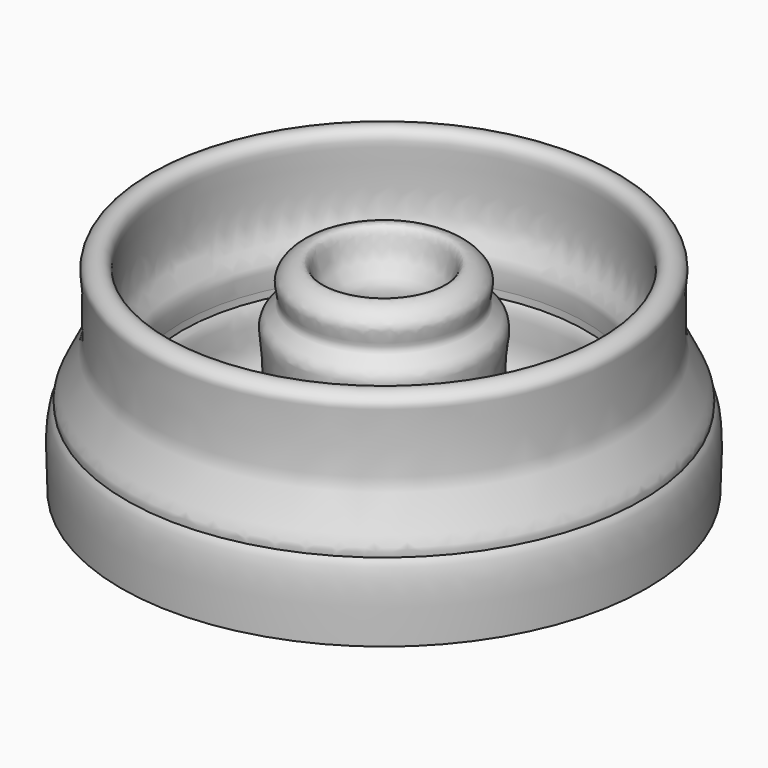
from build123d import *


with BuildPart() as f1:
    # F0 (on Front) → F1 (revolve)
    with BuildSketch(Plane.XZ):
        with BuildLine():
            add(Edge.make_bspline(
                [(-5.5100140162, 0), (-7.4768554599, 1.6512499989), (-8.4868156211, 11.2822794795), (-11.6145699642, 16.211100514), (-14.0046197921, 17.3335876316)],
                knots=[0.0567445852, 0.0567445852, 0.0567445852, 0.0567445852, 0.1379704075, 0.2072796019, 0.2072796019, 0.2072796019, 0.2072796019], degree=3))
            add(Edge.make_bspline(
                [(-14.0046197921, 17.3335876316), (-16.264658586, 18.3950150553), (-19.3741295412, 18.430981238), (-21.3513057679, 17.5631716847)],
                knots=[0.2072796019, 0.2072796019, 0.2072796019, 0.2072796019, 0.2728185988, 0.2728185988, 0.2728185988, 0.2728185988], degree=3))
            add(Edge.make_bspline(
                [(-21.3513057679, 17.5631716847), (-22.9378846487, 16.8668006222), (-24.856551537, 14.0064203945), (-25.3428790843, 6.7308083338), (-27.5189999089, 1.7281130761), (-30.8207862539, 0.4264153255), (-32.6009168711, 1.22e-08)],
                knots=[0.2728185988, 0.2728185988, 0.2728185988, 0.2728185988, 0.3254101619, 0.390496916, 0.4452692569, 0.4997726035, 0.4997726035, 0.4997726035, 0.4997726035], degree=3))
            add(Edge.make_bspline(
                [(-32.6009168435, 0), (-23.5706158992, 0), (-14.5403149549, 0), (-5.5100140107, 0)],
                knots=[25.9429850471, 25.9429850471, 25.9429850471, 25.9429850471, 53.0338878798, 53.0338878798, 53.0338878798, 53.0338878798], degree=3))
        make_face()
        with BuildLine():
            add(Edge.make_bspline(
                [(-14.0046197921, 17.3335876316), (-16.264658586, 18.3950150553), (-19.3741295412, 18.430981238), (-21.3513057679, 17.5631716847)],
                knots=[0.2072796019, 0.2072796019, 0.2072796019, 0.2072796019, 0.2728185988, 0.2728185988, 0.2728185988, 0.2728185988], degree=3))
            add(Edge.make_bspline(
                [(-21.3513057679, 17.5631716847), (-21.1820220673, 21.0577877247), (-20.8801300759, 27.2899092584), (-22.6799382537, 34.1653744535), (-17.1221063441, 36.9227227126), (-20.7290149123, 42.3952693374), (-12.6347622732, 47.302902282), (-12.7254316197, 39.345986815), (-7.9522904735, 35.8953625402), (-10.1102283491, 28.7576830255), (-7.0596366051, 15.4205940348), (-12.0270388133, 16.7888635267), (-14.0046197921, 17.3335876316)],
                knots=[0, 0, 0, 0, 0.1262257386, 0.2251045993, 0.3085069257, 0.3957592528, 0.4903294159, 0.583105022, 0.673312871, 0.780958545, 0.9127970322, 1, 1, 1, 1], degree=3))
        make_face()
    revolve(axis=Axis((0, 0, 38.2831208408), (0, 0, 1)))


with BuildPart() as f1b:
    # F0 (on Front) → F1, piece 2 (revolve)
    with BuildSketch(Plane.XZ):
        with BuildLine():
            add(Edge.make_bspline(
                [(-58.5439018905, 0), (-51.7329126534, 0), (-44.9219234162, 0), (-38.1109341791, 0)],
                knots=[0, 0, 0, 0, 20.4329677115, 20.4329677115, 20.4329677115, 20.4329677115], degree=3))
            add(Edge.make_bspline(
                [(-38.1109341979, 0), (-39.7350614236, 0.6328310893), (-42.3709629032, 3.5674251118), (-44.497911567, 8.512945314), (-43.4937968549, 15.0815158027), (-44.9984520674, 16.8744195253)],
                knots=[0.5565172055, 0.5565172055, 0.5565172055, 0.5565172055, 0.6120735986, 0.6692323198, 0.7381048965, 0.7381048965, 0.7381048965, 0.7381048965], degree=3))
            add(Edge.make_bspline(
                [(-44.9984520674, 16.8744195253), (-46.4682072785, 18.6257374135), (-52.6748450805, 18.6928178626), (-56.4195166036, 18.0445218661), (-57.3959834874, 16.8744195253)],
                knots=[0.7381048965, 0.7381048965, 0.7381048965, 0.7381048965, 0.8053799955, 0.8598764036, 0.8598764036, 0.8598764036, 0.8598764036], degree=3))
            add(Edge.make_bspline(
                [(-57.3959834874, 16.8744195253), (-58.5065944281, 15.5435720761), (-58.971992813, 9.9615017872), (-58.697162445, 3.5663108174), (-58.5439018905, 0)],
                knots=[0.8598764036, 0.8598764036, 0.8598764036, 0.8598764036, 0.9218593627, 1, 1, 1, 1], degree=3))
        make_face()
        with BuildLine():
            add(Edge.make_bspline(
                [(-44.9984520674, 16.8744195253), (-46.4682072785, 18.6257374135), (-52.6748450805, 18.6928178626), (-56.4195166036, 18.0445218661), (-57.3959834874, 16.8744195253)],
                knots=[0.7381048965, 0.7381048965, 0.7381048965, 0.7381048965, 0.8053799955, 0.8598764036, 0.8598764036, 0.8598764036, 0.8598764036], degree=3))
            add(Edge.make_bspline(
                [(-44.9984520674, 18.4815078974), (-44.9984520674, 17.9458117733), (-44.9984520674, 17.4101156493), (-44.9984520674, 16.8744195253)],
                knots=[0, 0, 0, 0, 1.6070883721, 1.6070883721, 1.6070883721, 1.6070883721], degree=3))
            add(Edge.make_bspline(
                [(-57.3959834874, 16.8744195253), (-57.4715446562, 17.3499237875), (-57.6848422564, 18.6921994511), (-54.9401189391, 23.4840896745), (-51.9408575122, 29.3763854334), (-52.8208897576, 35.1752529667), (-52.2423948178, 40.8160501854), (-53.4284694884, 44.8525009993), (-49.8042473471, 46.8159805052), (-47.0898142548, 45.1735042208), (-47.5753866113, 40.3334642214), (-48.4768776708, 28.2128829532), (-44.2823912341, 24.1291973687), (-44.7602116927, 20.3605488851), (-44.9984520674, 18.4815078974)],
                knots=[0, 0, 0, 0, 0.0480091479, 0.1355224673, 0.2335006939, 0.3242294406, 0.4149581578, 0.487541167, 0.5551750374, 0.6133988864, 0.694599797, 0.8254627536, 0.9129760599, 1, 1, 1, 1], degree=3))
        make_face()
    revolve(axis=Axis((0, 0, 38.2831208408), (0, 0, 1)))


with BuildPart() as f1c:
    # F0 (on Front) → F1, piece 3 (revolve)
    with BuildSketch(Plane.XZ):
        with BuildLine():
            add(Edge.make_bspline(
                [(-32.6009168711, 1.22e-08), (-34.4542490546, -0.4439501204), (-36.4520710376, -0.6463657239), (-38.1109341912, 7e-10)],
                knots=[0.4997726035, 0.4997726035, 0.4997726035, 0.4997726035, 0.5565172055, 0.5565172055, 0.5565172055, 0.5565172055], degree=3))
            add(Edge.make_bspline(
                [(-38.1109341791, 0), (-36.2742617339, 0), (-34.4375892887, 0), (-32.6009168435, 0)],
                knots=[20.4329677115, 20.4329677115, 20.4329677115, 20.4329677115, 25.9429850471, 25.9429850471, 25.9429850471, 25.9429850471], degree=3))
        make_face()
    revolve(axis=Axis((0, 0, 38.2831208408), (0, 0, 1)))


solid = Compound([f1.part, f1b.part, f1c.part])
